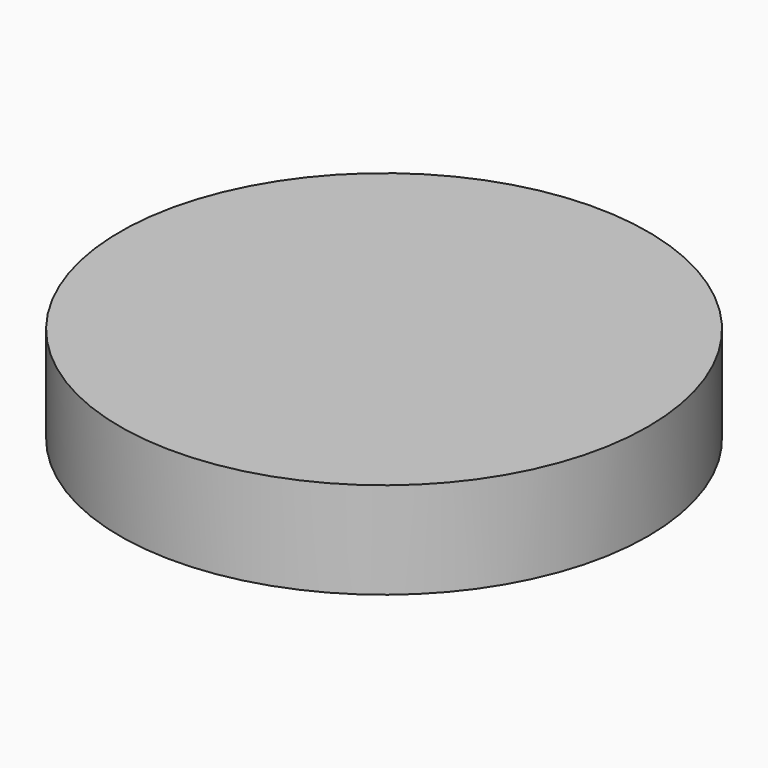
from build123d import *

# Parameters (mm, degrees)
F0_R     = 69.5520480584
F1_DEPTH = 25.4


# Not quite as in the source:
# - the program builds the solid bodies; features that only make, move or delete a surface that nothing else refers to are left out


with BuildPart() as f1:
    # F0 (on Top) → F1 (new body)
    with BuildSketch(Plane.XY):
        Circle(F0_R)
    extrude(amount=F1_DEPTH)


solid = f1.part
